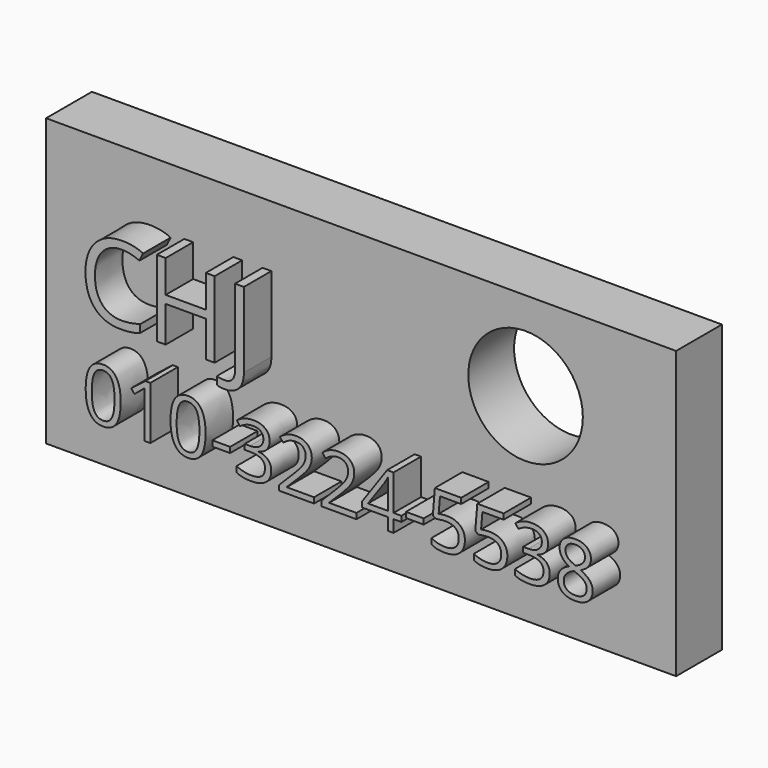
from build123d import *

# Parameters (mm, degrees)
F0_W           = 55
F0_H           = 25
F1_DEPTH       = 5
F2_TEXT_SIZE   = 9.3203883495
F2_TEXT_SIZE_2 = 6.479044341
F3_DEPTH       = 3
F4_R           = 5
F5_DEPTH       = 25


# Not quite as in the source:
# - Text() gives the source's letters only with a copy of the font that has no kerning and outlines rounded to 1/6400 em; it was checked with that copy


with BuildPart() as f1:
    # F0 (on Front) → F1 (new body)
    with BuildSketch(Plane.XZ):
        with Locations((27.5, 12.5)):
            Rectangle(F0_W, F0_H)
    extrude(amount=F1_DEPTH)

    # F2 (on face) → F3 (join)
    with BuildSketch(Plane.XZ.offset(5)):
        with Locations((5.2713023814, 12.993720243)):
            Text('CHJ', F2_TEXT_SIZE, font='Open Sans', text_align=(TextAlign.LEFT, TextAlign.BOTTOM))
        with Locations((5.5342703126, 4.9899197184)):
            Text('010-3224-5538', F2_TEXT_SIZE_2, font='Open Sans', text_align=(TextAlign.LEFT, TextAlign.BOTTOM))
    extrude(amount=F3_DEPTH)

    # F4 (on face) → F5 (cut)
    with BuildSketch(Plane.XZ.offset(5)):
        with Locations((41.8578022142, 17.2602945289)):
            Circle(F4_R)
    extrude(amount=-F5_DEPTH, mode=Mode.SUBTRACT)


solid = f1.part
